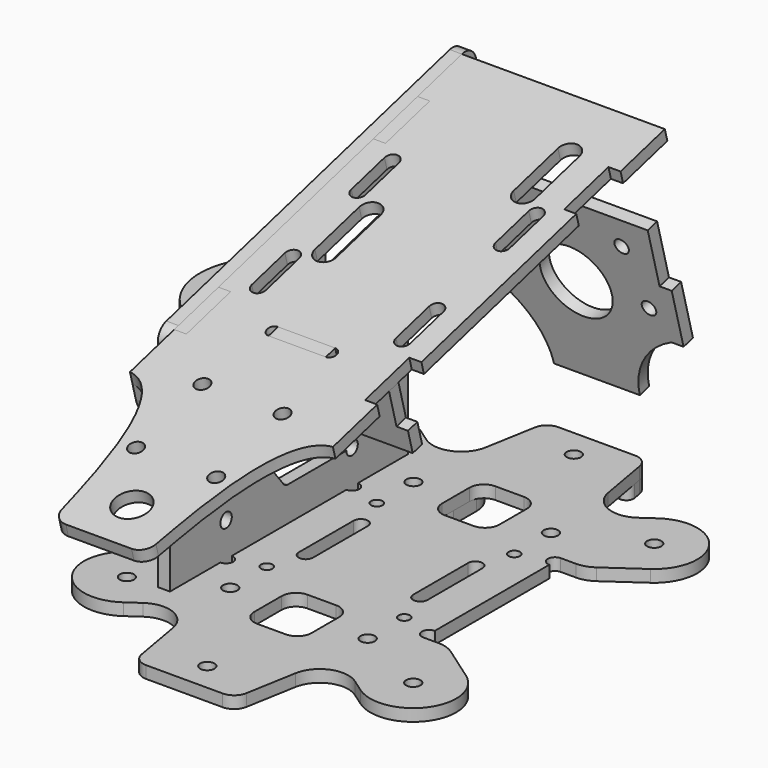
from build123d import *

# Parameters (mm, degrees)
F5_DEPTH  = 2.6924
F6_R      = 1.5875
F6_R_2    = 3.175
F7_DEPTH  = 2.6924
F9_DEPTH  = 2.6924
F10_R     = 1.27
F10_R_2   = 1.5875
F11_DEPTH = 2.6924
F13_DEPTH = 2.6924
F14_R     = 1.5875
F15_DEPTH = 2.6924
F17_DEPTH = 2.6924
F18_R     = 1.5875
F19_DEPTH = 2.6924
F21_DEPTH = 2.6924
F22_R     = 3.81
F22_R_2   = 1.5875
F23_DEPTH = 2.6924
F25_DEPTH = 2.6924
F26_R     = 7.9375
F26_R_2   = 1.5875
F27_DEPTH = 2.6924
F29_DEPTH = 2.6924
F31_DEPTH = 2.6924
F32_D     = 3.175


# Not quite as in the source:
# - ends of sketch curves that miss each other by under 0.0002 mm in the source are joined


with BuildPart() as f5:
    # F3 (on Top) → F5 (new body)
    with BuildSketch(Plane.XY):
        with BuildLine():
            ThreePointArc((-60.2589606516, 64.9933956321), (-63.310101302, 68.0165066287), (-65.1790406289, 71.8837698934))
            ThreePointArc((-65.1790406289, 71.8837698934), (-93.4387052306, 76.5982249442), (-79.343192071, 51.6552652442))
            ThreePointArc((-79.343192071, 51.6552652442), (-75.069938422, 51.2217186862), (-71.1855917641, 49.3885491883))
            Line((-71.1855917641, 49.3885491883), (-29.4977162748, 20.1983845188))
            ThreePointArc((-29.4977162748, 20.1983845188), (-27.7649877308, 19.3438973627), (-25.8555059039, 19.05))
            Line((-25.8555059039, 19.05), (-12.7, 19.05))
            ThreePointArc((-12.7, 19.05), (-8.2098719395, 20.9098719395), (-6.35, 25.4))
            Line((-6.35, 25.4), (-6.35, 31.75))
            ThreePointArc((-6.35, 31.75), (-8.2098719395, 36.2401280605), (-12.7, 38.1))
            Line((-12.7, 38.1), (-19.8490639758, 38.1))
            ThreePointArc((-19.8490639758, 38.1), (-21.7585458026, 38.3938973627), (-23.4912743466, 39.2483845188))
            Line((-23.4912743466, 39.2483845188), (-60.2589606516, 64.9933956321))
        make_face()
    extrude(amount=-F5_DEPTH)

    # F6 (on face) → F7 (cut, through all)
    with BuildSketch(Plane.XY):
        with Locations((-31.75, 33.4033285193)):
            Circle(F6_R)
        with BuildLine():
            Line((-76.879385229, 73.5820019586), (-77.4900125345, 72.8542846736))
            ThreePointArc((-77.4900125345, 72.8542846736), (-77.3432598672, 71.1768940107), (-75.6658692043, 71.323646678))
            Line((-75.6658692043, 71.323646678), (-75.0552418988, 72.051363963))
            ThreePointArc((-75.0552418988, 72.051363963), (-74.5155872578, 72.2365793621), (-74.0762700965, 72.6006292317))
            Line((-74.0762700965, 72.6006292317), (-73.112088682, 73.7496958963))
            ThreePointArc((-73.112088682, 73.7496958963), (-73.3077589051, 75.9862167802), (-75.5442797889, 75.7905465571))
            Line((-75.5442797889, 75.7905465571), (-76.5084612035, 74.6414798924))
            ThreePointArc((-76.5084612035, 74.6414798924), (-76.7906937131, 74.1456203496), (-76.879385229, 73.5820019586))
        make_face()
        with BuildLine():
            Line((-74.345363586, 63.9374177186), (-75.073080871, 64.5480450241))
            ThreePointArc((-75.073080871, 64.5480450241), (-76.7504715339, 64.4012923568), (-76.6037188666, 62.7239016939))
            Line((-76.6037188666, 62.7239016939), (-75.8760015816, 62.1132743884))
            ThreePointArc((-75.8760015816, 62.1132743884), (-75.6907861825, 61.5736197473), (-75.3267363129, 61.1343025861))
            Line((-75.3267363129, 61.1343025861), (-74.1776696482, 60.1701211716))
            ThreePointArc((-74.1776696482, 60.1701211716), (-71.9411487644, 60.3657913947), (-72.1368189875, 62.6023122785))
            Line((-72.1368189875, 62.6023122785), (-73.2858856522, 63.566493693))
            ThreePointArc((-73.2858856522, 63.566493693), (-73.781745195, 63.8487262026), (-74.345363586, 63.9374177186))
        make_face()
        with Locations((-80.4346665275, 67.4926990171)):
            Circle(F6_R_2)
        with BuildLine():
            Line((-86.523969469, 71.0479803156), (-85.796252184, 70.4373530101))
            ThreePointArc((-85.796252184, 70.4373530101), (-84.1188615211, 70.5841056774), (-84.2656141884, 72.2614963403))
            Line((-84.2656141884, 72.2614963403), (-84.9933314734, 72.8721236457))
            ThreePointArc((-84.9933314734, 72.8721236457), (-85.1785468725, 73.4117782868), (-85.5425967421, 73.851095448))
            Line((-85.5425967421, 73.851095448), (-86.6916634067, 74.8152768626))
            ThreePointArc((-86.6916634067, 74.8152768626), (-88.9281842906, 74.6196066395), (-88.7325140675, 72.3830857557))
            Line((-88.7325140675, 72.3830857557), (-87.5834474028, 71.4189043411))
            ThreePointArc((-87.5834474028, 71.4189043411), (-87.08758786, 71.1366718315), (-86.523969469, 71.0479803156))
        make_face()
        with BuildLine():
            Line((-83.989947826, 61.4033960756), (-83.3793205205, 62.1311133606))
            ThreePointArc((-83.3793205205, 62.1311133606), (-83.5260731878, 63.8085040235), (-85.2034638507, 63.6617513562))
            Line((-85.2034638507, 63.6617513562), (-85.8140911562, 62.9340340711))
            ThreePointArc((-85.8140911562, 62.9340340711), (-86.3537457972, 62.7488186721), (-86.7930629584, 62.3847688025))
            Line((-86.7930629584, 62.3847688025), (-87.757244373, 61.2357021378))
            ThreePointArc((-87.757244373, 61.2357021378), (-87.5615741499, 58.999181254), (-85.3250532661, 59.1948514771))
            Line((-85.3250532661, 59.1948514771), (-84.3608718515, 60.3439181418))
            ThreePointArc((-84.3608718515, 60.3439181418), (-84.0786393419, 60.8397776846), (-83.989947826, 61.4033960756))
        make_face()
        with Locations((-15.24, 25.4)):
            Circle(F6_R)
    extrude(amount=-F7_DEPTH, mode=Mode.SUBTRACT)


with BuildPart() as f9:
    # F8 (on Top) → F9 (new body)
    with BuildSketch(Plane.XY):
        with BuildLine():
            ThreePointArc((-26.2866844438, 41.2057517412), (-39.5524232219, 38.8666440756), (-37.2133155562, 25.6009052975))
            Line((-37.2133155562, 25.6009052975), (-29.4977162748, 20.1983845188))
            ThreePointArc((-29.4977162748, 20.1983845188), (-27.7649877308, 19.3438973627), (-25.8555059039, 19.05))
            Line((-25.8555059039, 19.05), (-22.5044, 19.05))
            ThreePointArc((-22.5044, 19.05), (-20.9169, 17.4625), (-22.5044, 15.875))
            Line((-22.5044, 15.875), (-22.5044, 0))
            Line((-22.5044, 0), (-22.5044, -15.875))
            ThreePointArc((-22.5044, -15.875), (-20.9169, -17.4625), (-22.5044, -19.05))
            Line((-22.5044, -19.05), (-25.8555059039, -19.05))
            ThreePointArc((-25.8555059039, -19.05), (-27.7649877308, -19.3438973627), (-29.4977162748, -20.1983845188))
            Line((-29.4977162748, -20.1983845188), (-37.2133155562, -25.6009052975))
            ThreePointArc((-37.2133155562, -25.6009052975), (-39.5524232219, -38.8666440756), (-26.2866844438, -41.2057517412))
            Line((-26.2866844438, -41.2057517412), (-23.4912743466, -39.2483845188))
            ThreePointArc((-23.4912743466, -39.2483845188), (-17.4190241803, -38.5833649686), (-13.5955347442, -43.3473340718))
            Line((-13.5955347442, -43.3473340718), (-11.6243756222, -54.5263329641))
            ThreePointArc((-11.6243756222, -54.5263329641), (-10.5384616671, -56.4071911069), (-8.4976110063, -57.15))
            Line((-8.4976110063, -57.15), (0, -57.15))
            Line((0, -57.15), (8.4976110063, -57.15))
            ThreePointArc((8.4976110063, -57.15), (10.5384616671, -56.4071911069), (11.6243756222, -54.5263329641))
            Line((11.6243756222, -54.5263329641), (13.5955347442, -43.3473340718))
            ThreePointArc((13.5955347442, -43.3473340718), (17.4190241803, -38.5833649686), (23.4912743466, -39.2483845188))
            Line((23.4912743466, -39.2483845188), (26.2866844438, -41.2057517412))
            ThreePointArc((26.2866844438, -41.2057517412), (39.5524232219, -38.8666440756), (37.2133155562, -25.6009052975))
            Line((37.2133155562, -25.6009052975), (29.4977162748, -20.1983845188))
            ThreePointArc((29.4977162748, -20.1983845188), (27.7649877308, -19.3438973627), (25.8555059039, -19.05))
            Line((25.8555059039, -19.05), (22.5044, -19.05))
            ThreePointArc((22.5044, -19.05), (20.9169, -17.4625), (22.5044, -15.875))
            Line((22.5044, -15.875), (22.5044, 0))
            Line((22.5044, 0), (22.5044, 15.875))
            ThreePointArc((22.5044, 15.875), (20.9169, 17.4625), (22.5044, 19.05))
            Line((22.5044, 19.05), (25.8555059039, 19.05))
            ThreePointArc((25.8555059039, 19.05), (27.7649877308, 19.3438973627), (29.4977162748, 20.1983845188))
            Line((29.4977162748, 20.1983845188), (37.2133155562, 25.6009052975))
            ThreePointArc((37.2133155562, 25.6009052975), (39.5524232219, 38.8666440756), (26.2866844438, 41.2057517412))
            Line((26.2866844438, 41.2057517412), (23.4912743466, 39.2483845188))
            ThreePointArc((23.4912743466, 39.2483845188), (17.4190241803, 38.5833649686), (13.5955347442, 43.3473340718))
            Line((13.5955347442, 43.3473340718), (11.6243756222, 54.5263329641))
            ThreePointArc((11.6243756222, 54.5263329641), (10.5384616671, 56.4071911069), (8.4976110063, 57.15))
            Line((8.4976110063, 57.15), (0, 57.15))
            Line((0, 57.15), (-8.4976110063, 57.15))
            ThreePointArc((-8.4976110063, 57.15), (-10.5384616671, 56.4071911069), (-11.6243756222, 54.5263329641))
            Line((-11.6243756222, 54.5263329641), (-13.5955347442, 43.3473340718))
            ThreePointArc((-13.5955347442, 43.3473340718), (-17.4190241803, 38.5833649686), (-23.4912743466, 39.2483845188))
            Line((-23.4912743466, 39.2483845188), (-26.2866844438, 41.2057517412))
        make_face()
    extrude(amount=F9_DEPTH)

    # F10 (on Top) → F11 (cut, through all)
    with BuildSketch(Plane.XY):
        with Locations((-15.25, 15.25)):
            Circle(F10_R)
        with BuildLine():
            Line((-3.175, 19.05), (0, 19.05))
            Line((0, 19.05), (3.175, 19.05))
            ThreePointArc((3.175, 19.05), (5.4200640303, 19.9799359697), (6.35, 22.225))
            Line((6.35, 22.225), (6.35, 29.845))
            ThreePointArc((6.35, 29.845), (5.4200640303, 32.0900640303), (3.175, 33.02))
            Line((3.175, 33.02), (0, 33.02))
            Line((0, 33.02), (-3.175, 33.02))
            ThreePointArc((-3.175, 33.02), (-5.4200640303, 32.0900640303), (-6.35, 29.845))
            Line((-6.35, 29.845), (-6.35, 22.225))
            ThreePointArc((-6.35, 22.225), (-5.4200640303, 19.9799359697), (-3.175, 19.05))
        make_face()
        with Locations((-15.24, 25.4)):
            Circle(F10_R_2)
        with Locations((-31.75, 33.4033285193)):
            Circle(F10_R_2)
        with Locations((31.75, 33.4033285193)):
            Circle(F10_R_2)
        with Locations((15.24, 25.4)):
            Circle(F10_R_2)
        with Locations((15.25, 15.25)):
            Circle(F10_R)
        with BuildLine():
            Line((0, -33.02), (3.175, -33.02))
            ThreePointArc((3.175, -33.02), (5.4200640303, -32.0900640303), (6.35, -29.845))
            Line((6.35, -29.845), (6.35, -22.225))
            ThreePointArc((6.35, -22.225), (5.4200640303, -19.9799359697), (3.175, -19.05))
            Line((3.175, -19.05), (0, -19.05))
            Line((0, -19.05), (-3.175, -19.05))
            ThreePointArc((-3.175, -19.05), (-5.4200640303, -19.9799359697), (-6.35, -22.225))
            Line((-6.35, -22.225), (-6.35, -29.845))
            ThreePointArc((-6.35, -29.845), (-5.4200640303, -32.0900640303), (-3.175, -33.02))
            Line((-3.175, -33.02), (0, -33.02))
        make_face()
        with Locations((-31.75, -33.4033285193)):
            Circle(F10_R_2)
        with Locations((31.75, -33.4033285193)):
            Circle(F10_R_2)
        with Locations((15.24, -25.4)):
            Circle(F10_R_2)
        with Locations((-15.24, -25.4)):
            Circle(F10_R_2)
        with Locations((15.25, -15.25)):
            Circle(F10_R)
        with Locations((-15.25, -15.25)):
            Circle(F10_R)
        with BuildLine():
            Line((-11.1125, -7.62), (-11.1125, 7.62))
            ThreePointArc((-11.1125, 7.62), (-12.7, 9.2075), (-14.2875, 7.62))
            Line((-14.2875, 7.62), (-14.2875, -7.62))
            ThreePointArc((-14.2875, -7.62), (-12.7, -9.2075), (-11.1125, -7.62))
        make_face()
        with BuildLine():
            ThreePointArc((14.2875, 7.62), (12.7, 9.2075), (11.1125, 7.62))
            Line((11.1125, 7.62), (11.1125, -7.62))
            ThreePointArc((11.1125, -7.62), (12.7, -9.2075), (14.2875, -7.62))
            Line((14.2875, -7.62), (14.2875, 7.62))
        make_face()
        with Locations((0, 50.8)):
            Circle(F10_R_2)
        with Locations((0, -50.8)):
            Circle(F10_R_2)
    extrude(amount=F11_DEPTH, mode=Mode.SUBTRACT)


with BuildPart() as f13:
    # F12 (on face) → F13 (new body)
    with BuildSketch(Plane(origin=(-22.5044, 0, 0), x_dir=(0, -1, 0), z_dir=(-1, 0, 0))):
        with BuildLine():
            Line((-33.02, 28.1312823648), (-33.02, 2.6924))
            Line((-33.02, 2.6924), (-19.05, 2.6924))
            Line((-19.05, 2.6924), (-19.05, -2.3876))
            Line((-19.05, -2.3876), (19.05, -2.3876))
            Line((19.05, -2.3876), (19.05, 2.6924))
            Line((19.05, 2.6924), (33.02, 2.6924))
            Line((33.02, 2.6924), (33.02, 50.6147259851))
            ThreePointArc((33.02, 50.6147259851), (32.3638968554, 52.5475435222), (30.6667504682, 53.6815404836))
            Line((30.6667504682, 53.6815404836), (-47.898190218, 74.7329528939))
            ThreePointArc((-47.898190218, 74.7329528939), (-50.3074406862, 74.4157690524), (-51.7867551847, 72.4878888636))
            Line((-51.7867551847, 72.4878888636), (-57.5390084621, 51.0201873743))
            ThreePointArc((-57.5390084621, 51.0201873743), (-56.9046407792, 46.2016864379), (-53.0488804015, 43.243057441))
            Line((-53.0488804015, 43.243057441), (-42.4329981272, 40.3985403586))
            ThreePointArc((-42.4329981272, 40.3985403586), (-35.6444125783, 35.8625525132), (-33.02, 28.1312823648))
        make_face()
    extrude(amount=F13_DEPTH)

    # F14 (on face) → F15 (cut, through all)
    with BuildSketch(Plane.YZ.offset(-22.5044)):
        with Locations((44.45, 50.8)):
            Circle(F14_R)
        with Locations((-25.3492903722, 41.4148221362)):
            Circle(F14_R)
        with Locations((-24.2657108518, 35.3671265758)):
            Circle(F14_R)
        with Locations((-22.6591632802, 29.4368845007)):
            Circle(F14_R)
        with Locations((-20.5418744543, 23.6692286341)):
            Circle(F14_R)
        with Locations((-17.9299582207, 18.1080543195)):
            Circle(F14_R)
        with Locations((26.19375, 16.6624)):
            Circle(F14_R)
        with BuildLine():
            ThreePointArc((-2.5970108504, 49.3229533392), (-3.2372022504, 50.5475961441), (-4.5946042997, 50.806545376))
            Line((-4.5946042997, 50.806545376), (-15.1163610063, 47.9872491635))
            ThreePointArc((-15.1163610063, 47.9872491635), (-15.9995170023, 47.3734284656), (-16.2887184948, 46.3375216845))
            ThreePointArc((-16.2887184948, 46.3375216845), (-11.7789965568, 27.4032997343), (-1.5261312748, 10.8587808133))
            ThreePointArc((-1.5261312748, 10.8587808133), (-0.9862556185, 10.4554393811), (-0.327704352, 10.3124))
            Line((-0.327704352, 10.3124), (15.875, 10.3124))
            ThreePointArc((15.875, 10.3124), (18.2116251172, 8.9127686882), (18.3429909403, 11.6333435848))
            ThreePointArc((18.3429909403, 11.6333435848), (3.3038661827, 27.9395851157), (-2.5970108504, 49.3229533392))
        make_face()
        with BuildLine():
            ThreePointArc((30.4371196651, 49.9881455585), (31.0190074216, 50.7457007385), (31.0608316563, 51.7000245542))
            Line((31.0608316563, 51.7000245542), (29.3066153674, 58.2468488718))
            ThreePointArc((29.3066153674, 58.2468488718), (28.5669581182, 59.2107889662), (27.3623328841, 59.369380887))
            Line((27.3623328841, 59.369380887), (11.3720982578, 55.0848104321))
            ThreePointArc((11.3720982578, 55.0848104321), (10.5652269125, 54.5698576582), (10.2010745467, 53.6846397292))
            ThreePointArc((10.2010745467, 53.6846397292), (11.2918078183, 41.7532142553), (16.4118071832, 30.9211221483))
            ThreePointArc((16.4118071832, 30.9211221483), (18.0881532366, 30.2982680708), (19.2806159339, 31.6309780948))
            ThreePointArc((19.2806159339, 31.6309780948), (22.9289220086, 41.982479569), (30.4371196651, 49.9881455585))
        make_face()
        with Locations((-17.4625, 10.3124)):
            Circle(F14_R)
    extrude(amount=-F15_DEPTH, mode=Mode.SUBTRACT)


with BuildPart() as f17:
    # F16 (on face) → F17 (new body)
    with BuildSketch(Plane(origin=(-22.5044, 0, 0), x_dir=(0, -1, 0), z_dir=(-1, 0, 0))):
        with BuildLine():
            Line((-36.3277766212, 68.8452923264), (-48.595034615, 72.1322941992))
            Line((-48.595034615, 72.1322941992), (-53.6504434954, 53.2652514046))
            ThreePointArc((-53.6504434954, 53.2652514046), (-53.3529871711, 47.414376803), (-49.6875592646, 42.8442726323))
            Line((-49.6875592646, 42.8442726323), (-53.1000307563, 30.108755646))
            Line((-53.1000307563, 30.108755646), (-50.2022532774, 29.3322985107))
            ThreePointArc((-50.2022532774, 29.3322985107), (-35.3835337587, 30.5083806734), (-24.620859535, 40.7622804673))
            ThreePointArc((-24.620859535, 40.7622804673), (-21.5458097568, 43.6919661227), (-17.3118898943, 44.0279895977))
            Line((-17.3118898943, 44.0279895977), (23.6710072188, 33.0466554128))
            ThreePointArc((23.6710072188, 33.0466554128), (26.1433494758, 32.88460954), (28.4895081552, 33.6810230957))
            Line((28.4895081552, 33.6810230957), (39.4880307833, 40.0310230957))
            ThreePointArc((39.4880307833, 40.0310230957), (41.3508244941, 41.6646493355), (42.4466597802, 43.8867834733))
            Line((42.4466597802, 43.8867834733), (43.409400339, 47.4797801532))
            Line((43.409400339, 47.4797801532), (31.1421423451, 50.766782026))
            Line((31.1421423451, 50.766782026), (31.8389867422, 53.3674407207))
            Line((31.8389867422, 53.3674407207), (19.5717287483, 56.6544425935))
            Line((19.5717287483, 56.6544425935), (18.8748843513, 54.0537838988))
            Line((18.8748843513, 54.0537838988), (-24.0605186273, 65.5582904536))
            Line((-24.0605186273, 65.5582904536), (-23.3636742303, 68.1589491483))
            Line((-23.3636742303, 68.1589491483), (-35.6309322241, 71.4459510211))
            Line((-35.6309322241, 71.4459510211), (-36.3277766212, 68.8452923264))
        make_face()
    extrude(amount=-F17_DEPTH)

    # F18 (on face) → F19 (cut, through all)
    with BuildSketch(Plane(origin=(-22.5044, 0, 0), x_dir=(0, -1, 0), z_dir=(-1, 0, 0))):
        Polygon((-46.8994897428, 53.2494897428), (-47.796065215, 49.9034245278), (-45.3465754722, 47.453934785), (-42.0005102572, 48.3505102572), (-41.103934785, 51.6965754722), (-43.5534245278, 54.146065215), align=None)
        with BuildLine():
            Line((26.2458658444, 44.7608873511), (22.8998006294, 43.864311879))
            Line((22.8998006294, 43.864311879), (23.1089132679, 44.6447308703))
            ThreePointArc((23.1089132679, 44.6447308703), (22.1570061191, 46.2934824161), (20.5082545732, 45.3415752673))
            Line((20.5082545732, 45.3415752673), (19.1934538241, 40.4346720698))
            ThreePointArc((19.1934538241, 40.4346720698), (20.1453609729, 38.7859205239), (21.7941125188, 39.7378276727))
            Line((21.7941125188, 39.7378276727), (22.0032251573, 40.518246664))
            Line((22.0032251573, 40.518246664), (24.4527149, 38.0687569212))
            Line((24.4527149, 38.0687569212), (27.798780115, 38.9653323934))
            Line((27.798780115, 38.9653323934), (28.6953555872, 42.3113976084))
            Line((28.6953555872, 42.3113976084), (26.2458658444, 44.7608873511))
        make_face()
        with Locations((-46.8563080722, 35.0097589407)):
            Circle(F18_R)
        with BuildLine():
            Line((4.964125421, 51.2071567746), (-31.8376485606, 61.068162393))
            ThreePointArc((-31.8376485606, 61.068162393), (-35.7262135273, 58.8230983628), (-33.481149497, 54.9345333961))
            Line((-33.481149497, 54.9345333961), (3.3206244846, 45.0735277777))
            ThreePointArc((3.3206244846, 45.0735277777), (7.2091894513, 47.318591808), (4.964125421, 51.2071567746))
        make_face()
    extrude(amount=-F19_DEPTH, mode=Mode.SUBTRACT)


with BuildPart() as f21:
    # F20 (on face) → F21 (new body)
    with BuildSketch(Plane(origin=(0, -14.7778234795, 55.1515880507), x_dir=(1, 0, 0), z_dir=(0, -0.2588190451, 0.9659258263))):
        with BuildLine():
            Line((0, 65.6084104698), (-22.5044, 65.6084104698))
            Line((-22.5044, 65.6084104698), (-22.5044, 52.9084104698))
            Line((-22.5044, 52.9084104698), (-19.812, 52.9084104698))
            Line((-19.812, 52.9084104698), (-19.812, 40.2084104698))
            Line((-19.812, 40.2084104698), (-22.5044, 40.2084104698))
            Line((-22.5044, 40.2084104698), (-22.5044, -4.2415895302))
            Line((-22.5044, -4.2415895302), (-19.812, -4.2415895302))
            Line((-19.812, -4.2415895302), (-19.812, -16.9415895302))
            Line((-19.812, -16.9415895302), (-22.5044, -16.9415895302))
            Line((-22.5044, -16.9415895302), (-22.5044, -29.6415895302))
            add(Edge.make_bspline(
                [(-22.5044, -29.6415895302), (-12.3425725495, -30.7706814692), (-11.1950289472, -54.9875828189), (-10.4407699904, -64.8096883506)],
                knots=[0, 0, 0, 0, 35.6063112738, 35.6063112738, 35.6063112738, 35.6063112738], degree=3))
            ThreePointArc((-10.4407699904, -64.8096883506), (-9.4324945461, -66.8960169014), (-7.2750902903, -67.7415895302))
            Line((-7.2750902903, -67.7415895302), (0, -67.7415895302))
            Line((0, -67.7415895302), (7.2750902903, -67.7415895302))
            ThreePointArc((7.2750902903, -67.7415895302), (9.4324945461, -66.8960169014), (10.4407699904, -64.8096883506))
            add(Edge.make_bspline(
                [(22.5044, -29.6415895302), (12.3425725495, -30.7706814692), (11.1950289472, -54.9875828189), (10.4407699904, -64.8096883506)],
                knots=[0, 0, 0, 0, 35.6063112738, 35.6063112738, 35.6063112738, 35.6063112738], degree=3))
            Line((22.5044, -29.6415895302), (22.5044, -16.9415895302))
            Line((22.5044, -16.9415895302), (19.812, -16.9415895302))
            Line((19.812, -16.9415895302), (19.812, -4.2415895302))
            Line((19.812, -4.2415895302), (22.5044, -4.2415895302))
            Line((22.5044, -4.2415895302), (22.5044, 40.2084104698))
            Line((22.5044, 40.2084104698), (19.812, 40.2084104698))
            Line((19.812, 40.2084104698), (19.812, 52.9084104698))
            Line((19.812, 52.9084104698), (22.5044, 52.9084104698))
            Line((22.5044, 52.9084104698), (22.5044, 65.6084104698))
            Line((22.5044, 65.6084104698), (0, 65.6084104698))
        make_face()
    extrude(amount=F21_DEPTH)

    # F22 (on face) → F23 (cut, through all)
    with BuildSketch(Plane(origin=(0, -15.4746678765, 57.7522467454), x_dir=(1, 0, 0), z_dir=(0, -0.2588190451, 0.9659258263))):
        with BuildLine():
            Line((-14.4125, 27.5084104698), (-14.4125, 37.0334104698))
            ThreePointArc((-14.4125, 37.0334104698), (-16, 38.6209104698), (-17.5875, 37.0334104698))
            Line((-17.5875, 37.0334104698), (-17.5875, 27.5084104698))
            ThreePointArc((-17.5875, 27.5084104698), (-16, 25.9209104698), (-14.4125, 27.5084104698))
        make_face()
        with BuildLine():
            Line((-14.4125, -1.0665895302), (-14.4125, 8.4584104698))
            ThreePointArc((-14.4125, 8.4584104698), (-16, 10.0459104698), (-17.5875, 8.4584104698))
            Line((-17.5875, 8.4584104698), (-17.5875, -1.0665887242))
            ThreePointArc((-17.5875, -1.0665887242), (-16, -2.6540895302), (-14.4125, -1.0665895302))
        make_face()
        with BuildLine():
            Line((-8.61875, 11.6334104698), (-8.61875, 24.3334104698))
            ThreePointArc((-8.61875, 24.3334104698), (-11, 26.7146604698), (-13.38125, 24.3334104698))
            Line((-13.38125, 24.3334104698), (-13.38125, 11.6334104698))
            ThreePointArc((-13.38125, 11.6334104698), (-11, 9.2521604698), (-8.61875, 11.6334104698))
        make_face()
        with Locations((0, -58.2165895302)):
            Circle(F22_R)
        with BuildLine():
            ThreePointArc((17.5875, 37.0334104698), (16, 38.6209104698), (14.4125, 37.0334104698))
            Line((14.4125, 37.0334104698), (14.4125, 27.5084104698))
            ThreePointArc((14.4125, 27.5084104698), (16, 25.9209104698), (17.5875, 27.5084104698))
            Line((17.5875, 27.5084104698), (17.5875, 37.0334104698))
        make_face()
        with BuildLine():
            ThreePointArc((17.5875, 8.4584104698), (16, 10.0459104698), (14.4125, 8.4584104698))
            Line((14.4125, 8.4584104698), (14.4125, -1.0665895302))
            ThreePointArc((14.4125, -1.0665895302), (16, -2.6540895302), (17.5875, -1.0665895302))
            Line((17.5875, -1.0665895302), (17.5875, 8.4584104698))
        make_face()
        with BuildLine():
            Line((8.61875, 52.9084104698), (8.61875, 40.2084104698))
            ThreePointArc((8.61875, 40.2084104698), (11, 37.8271604698), (13.38125, 40.2084104698))
            Line((13.38125, 40.2084104698), (13.38125, 52.9084104698))
            ThreePointArc((13.38125, 52.9084104698), (11, 55.2896604698), (8.61875, 52.9084104698))
        make_face()
        with Locations((-8.89, -45.5165895302)):
            Circle(F22_R_2)
        with Locations((-8.89, -26.4665895302)):
            Circle(F22_R_2)
        with Locations((8.89, -26.4665895302)):
            Circle(F22_R_2)
        with Locations((8.89, -45.5165895302)):
            Circle(F22_R_2)
        with BuildLine():
            ThreePointArc((-6.35, -8.0744495302), (-7.6962, -9.4206495302), (-6.35, -10.7668495302))
            Line((-6.35, -10.7668495302), (6.35, -10.7668495302))
            ThreePointArc((6.35, -10.7668495302), (7.6962, -9.4206495302), (6.35, -8.0744495302))
            Line((6.35, -8.0744495302), (-6.35, -8.0744495302))
        make_face()
    extrude(amount=-F23_DEPTH, mode=Mode.SUBTRACT)


with BuildPart() as f25:
    # F24 (on face) → F25 (new body)
    with BuildSketch(Plane(origin=(0, 57.070192078, 15.2919118792), x_dir=(-1, 0, 0), z_dir=(0, 0.9659258263, 0.2588190451))):
        with BuildLine():
            Line((19.812, 28.0395254207), (19.812, 40.7395254207))
            Line((19.812, 40.7395254207), (0, 40.7395254207))
            Line((0, 40.7395254207), (-19.812, 40.7395254207))
            Line((-19.812, 40.7395254207), (-19.812, 28.0395254207))
            Line((-19.812, 28.0395254207), (-22.5044, 28.0395254207))
            Line((-22.5044, 28.0395254207), (-22.5044, 15.3395254207))
            Line((-22.5044, 15.3395254207), (-19.812, 15.3395254207))
            add(Edge.make_bspline(
                [(-19.812, 15.3395254207), (-13.462, 12.1645254207), (-9.525, 5.8145254207), (-9.525, -0.5354745793)],
                knots=[0, 0, 0, 0, 18.9166063024, 18.9166063024, 18.9166063024, 18.9166063024], degree=3))
            Line((-9.525, -0.5354745793), (0, -0.5354745793))
            Line((0, -0.5354745793), (9.525, -0.5354745793))
            add(Edge.make_bspline(
                [(19.812, 15.3395254207), (13.462, 12.1645254207), (9.525, 5.8145254207), (9.525, -0.5354745793)],
                knots=[0, 0, 0, 0, 18.9166063024, 18.9166063024, 18.9166063024, 18.9166063024], degree=3))
            Line((19.812, 15.3395254207), (22.5044, 15.3395254207))
            Line((22.5044, 15.3395254207), (22.5044, 28.0395254207))
            Line((22.5044, 28.0395254207), (19.812, 28.0395254207))
        make_face()
    extrude(amount=F25_DEPTH)

    # F26 (on face) → F27 (cut, through all)
    with BuildSketch(Plane(origin=(0, 59.6708507727, 15.9887562762), x_dir=(-1, 0, 0), z_dir=(0, 0.9659258263, 0.2588190451))):
        with Locations((0, 21.6895254207)):
            Circle(F26_R)
        with Locations((16.1544, 21.6895254207)):
            Circle(F26_R_2)
        with Locations((12.7, 34.3895254207)):
            Circle(F26_R_2)
        with Locations((-12.7, 34.3895254207)):
            Circle(F26_R_2)
        with Locations((-16.1544, 21.6895254207)):
            Circle(F26_R_2)
    extrude(amount=-F27_DEPTH, mode=Mode.SUBTRACT)


with BuildPart() as f29:
    # F28 (on face) → F29 (new body)
    with BuildSketch(Plane(origin=(0, -10.399978029, -2.7866657142), x_dir=(-1, 0, 0), z_dir=(0, 0.9659258263, 0.2588190451))):
        Polygon((6.35, 59.7895254207), (0, 59.7895254207), (-6.35, 59.7895254207), (-6.35, 57.0971254207), (-19.812, 57.0971254207), (-19.812, 49.1045254207), (-22.352, 49.1045254207), (-22.352, 44.0245254207), (0, 44.0245254207), (22.352, 44.0245254207), (22.352, 49.1045254207), (19.812, 49.1045254207), (19.812, 57.0971254207), (6.35, 57.0971254207), align=None)
    extrude(amount=F29_DEPTH)

    # F32 (through all)
    with Locations(Plane(origin=(0, -10.399978029, -2.7866657142), x_dir=(-1, 0, 0), z_dir=(0, -0.9659258263, -0.2588190451))):
        with Locations((-12.7, -50.3745254207), (12.7, -50.3745254207)):
            Hole(F32_D / 2)


with BuildPart() as f31:
    # F30 (on face) → F31 (new body)
    with BuildSketch(Plane(origin=(0, 0, 0), x_dir=(1, 0, 0), z_dir=(0, 0, -1))):
        with BuildLine():
            ThreePointArc((11.9529021425, -52.663166482), (11.605615388, -51.3670746696), (10.3895198346, -50.8))
            Line((10.3895198346, -50.8), (1.5875, -50.8))
            ThreePointArc((1.5875, -50.8), (0, -52.3875), (-1.5875, -50.8))
            Line((-1.5875, -50.8), (-10.3895198346, -50.8))
            ThreePointArc((-10.3895198346, -50.8), (-11.605615388, -51.3670746696), (-11.9529021425, -52.663166482))
            Line((-11.9529021425, -52.663166482), (-11.6243756222, -54.5263329641))
            ThreePointArc((-11.6243756222, -54.5263329641), (-10.5384616671, -56.4071911069), (-8.4976110063, -57.15))
            Line((-8.4976110063, -57.15), (8.4976110063, -57.15))
            ThreePointArc((8.4976110063, -57.15), (10.5384616671, -56.4071911069), (11.6243756222, -54.5263329641))
            Line((11.6243756222, -54.5263329641), (11.9529021425, -52.663166482))
        make_face()
    extrude(amount=F31_DEPTH)


solid = Compound([f5.part, f9.part, f13.part, f17.part, f21.part, f25.part, f29.part, f31.part])
